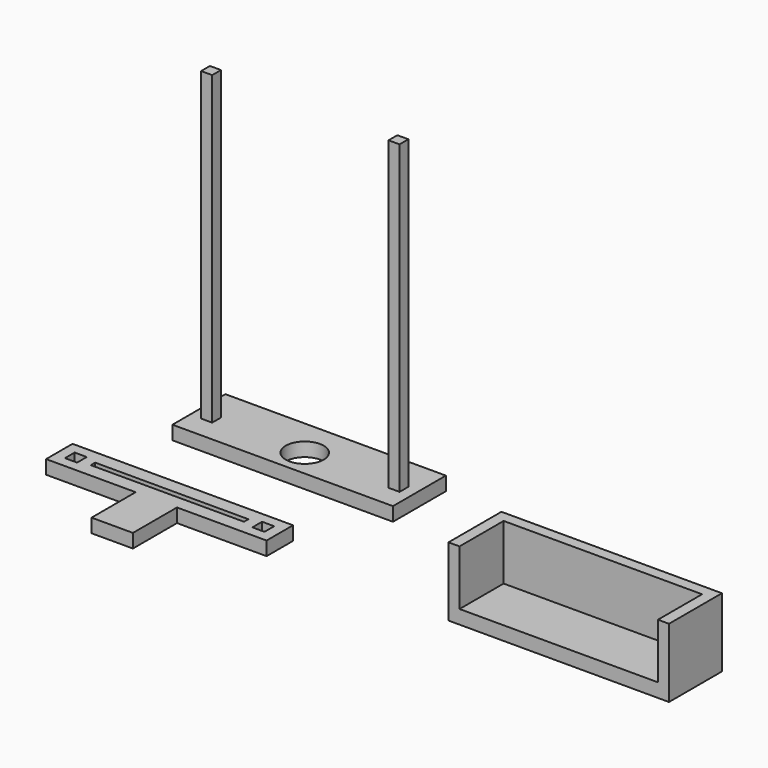
from build123d import *

# Parameters (mm, degrees)
F0_W     = 5.08
F0_H     = 5.08
F1_DEPTH = 147.32
F0_R     = 8.73125
F2_DEPTH = 6.35
F3_W     = 19.05
F3_H     = 25.4
F4_DEPTH = 6.35
F5_W     = 5.08
F5_H     = 5.08
F6_DEPTH = 31.75
F7_DEPTH = 25.4


# Not quite as in the source:
# - a feature names something its author has since deleted; it is built from what else it names


with BuildPart() as f1:
    # F0 (on Top) → F1 (new body)
    with BuildSketch(Plane.XY):
        with Locations((43.18, 0)):
            Rectangle(F0_W, F0_H)
    extrude(amount=F1_DEPTH)



with BuildPart() as f1b:
    # F0 (on Top) → F1, piece 2 (new body)
    with BuildSketch(Plane.XY):
        with Locations((-43.18, 0)):
            Rectangle(F0_W, F0_H)
    extrude(amount=F1_DEPTH)


with BuildPart() as f1_1:
    add(f1.part)

    add(f1b.part)  # F2 merges F1b
    # F0 (on Top) → F2 (join)
    with BuildSketch(Plane.XY):
        Polygon((45.72, 2.54), (45.72, 12.7), (-45.72, 12.7), (-45.72, 2.54), (-40.64, 2.54), (-40.64, -2.54), (-45.72, -2.54), (-45.72, -12.7), (45.72, -12.7), (45.72, -2.54), (40.64, -2.54), (40.64, 2.54), align=None)
        Circle(F0_R, mode=Mode.SUBTRACT)
        Polygon((-45.72, 12.7), (45.72, 12.7), (45.72, 2.54), (45.72, -2.54), (45.72, -12.7), (50.8, -12.7), (50.8, 17.78), (-50.8, 17.78), (-50.8, -12.7), (-45.72, -12.7), (-45.72, -2.54), (-45.72, 2.54), align=None)
    extrude(amount=F2_DEPTH)


with BuildPart() as f4:
    # F3 (on Top) → F4 (new body)
    with BuildSketch(Plane.XY):
        Polygon((-69.5630355358, -46.7925282216), (-69.5630355358, -62.0325282216), (-28.2880355358, -62.0325282216), (-9.2380355358, -62.0325282216), (32.0369644642, -62.0325282216), (32.0369644642, -46.7925282216), align=None)
        Polygon((-64.7370355358, -57.2065282216), (-64.7370355358, -51.6185282216), (-59.1490355358, -51.6185282216), (-54.0690355358, -51.6185282216), (-54.0690355358, -53.1425282216), (16.5429644642, -53.1425282216), (16.5429644642, -51.6185282216), (21.6229644642, -51.6185282216), (27.2109644642, -51.6185282216), (27.2109644642, -57.2065282216), (21.6229644642, -57.2065282216), (16.5429644642, -57.2065282216), (16.5429644642, -55.6825282216), (-54.0690355358, -55.6825282216), (-54.0690355358, -57.2065282216), (-59.1490355358, -57.2065282216), align=None, mode=Mode.SUBTRACT)
        with Locations((-18.7630355358, -74.7325282216)):
            Rectangle(F3_W, F3_H)
        Polygon((16.5429644642, -51.6185282216), (16.5429644642, -53.1425282216), (16.5429644642, -55.6825282216), (16.5429644642, -57.2065282216), (21.6229644642, -57.2065282216), (21.6229644642, -51.6185282216), align=None)
        Polygon((-54.0690355358, -51.6185282216), (-59.1490355358, -51.6185282216), (-59.1490355358, -57.2065282216), (-54.0690355358, -57.2065282216), (-54.0690355358, -55.6825282216), (-54.0690355358, -53.1425282216), align=None)
    extrude(amount=F4_DEPTH)


with BuildPart() as f6:
    # F5 (on Top) → F6 (new body)
    with BuildSketch(Plane.XY):
        Polygon((172.916882534, 2.5405777639), (172.916882534, 12.7005777639), (81.476882534, 12.7005777639), (81.476882534, 2.5405777639), (86.556882534, 2.5405777639), (86.556882534, -2.5394222361), (81.476882534, -2.5394222361), (81.476882534, -12.6994222361), (172.916882534, -12.6994222361), (172.916882534, -2.5394222361), (167.836882534, -2.5394222361), (167.836882534, 2.5405777639), align=None)
        Polygon((81.476882534, 12.7005777639), (172.916882534, 12.7005777639), (172.916882534, 2.5405777639), (172.916882534, -2.5394222361), (172.916882534, -12.6994222361), (177.996882534, -12.6994222361), (177.996882534, 17.7805777639), (76.396882534, 17.7805777639), (76.396882534, -12.6994222361), (81.476882534, -12.6994222361), (81.476882534, -2.5394222361), (81.476882534, 2.5405777639), align=None)
        with Locations((84.016882534, 0.0005777639)):
            Rectangle(F5_W, F5_H)
        with Locations((170.376882534, 0.0005777639)):
            Rectangle(F5_W, F5_H)
    extrude(amount=-F6_DEPTH)

    # F5 (on Top) → F7 (cut)
    with BuildSketch(Plane.XY):
        Polygon((172.916882534, 2.5405777639), (172.916882534, 12.7005777639), (81.476882534, 12.7005777639), (81.476882534, 2.5405777639), (86.556882534, 2.5405777639), (86.556882534, -2.5394222361), (81.476882534, -2.5394222361), (81.476882534, -12.6994222361), (172.916882534, -12.6994222361), (172.916882534, -2.5394222361), (167.836882534, -2.5394222361), (167.836882534, 2.5405777639), align=None)
        with Locations((170.376882534, 0.0005777639)):
            Rectangle(F5_W, F5_H)
        with Locations((84.016882534, 0.0005777639)):
            Rectangle(F5_W, F5_H)
    extrude(amount=-F7_DEPTH, mode=Mode.SUBTRACT)


solid = Compound([f1_1.part, f4.part, f6.part])
